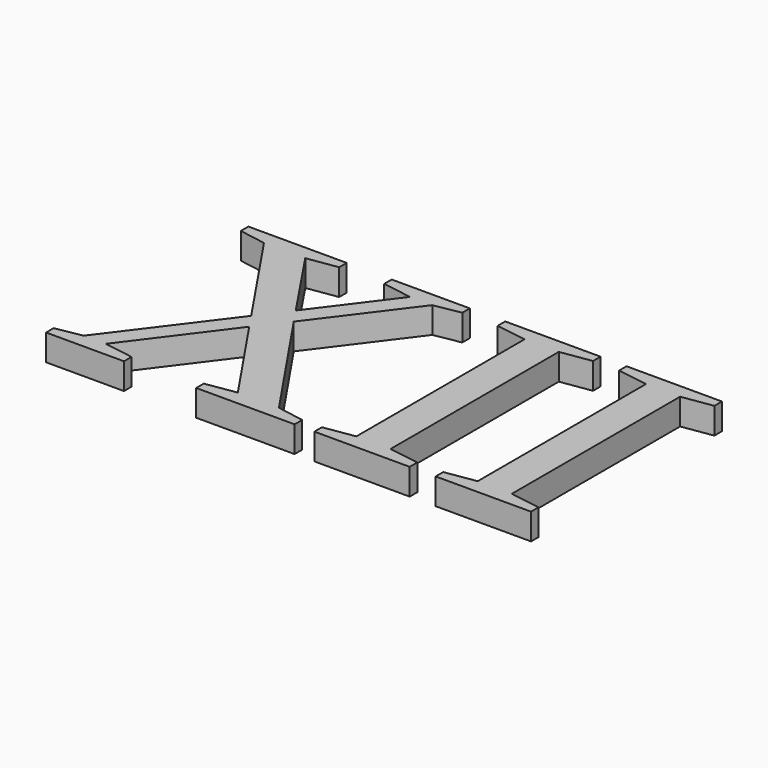
from build123d import *

# Parameters (mm, degrees)
F0_TEXT_SIZE = 35.2777777778
F1_DEPTH     = 2.54


# Not quite as in the source:
# - Text() gives the source's letters only with a copy of the font that has no kerning and outlines rounded to 1/6400 em; it was checked with that copy


with BuildPart() as f1:
    # F0 (on Top) → F1 (new body)
    with BuildSketch(Plane.XY):
        with Locations((0, 0)):
            Text('XII', F0_TEXT_SIZE, font='Tinos', text_align=(TextAlign.LEFT, TextAlign.BOTTOM))
    extrude(amount=F1_DEPTH)


solid = f1.part
